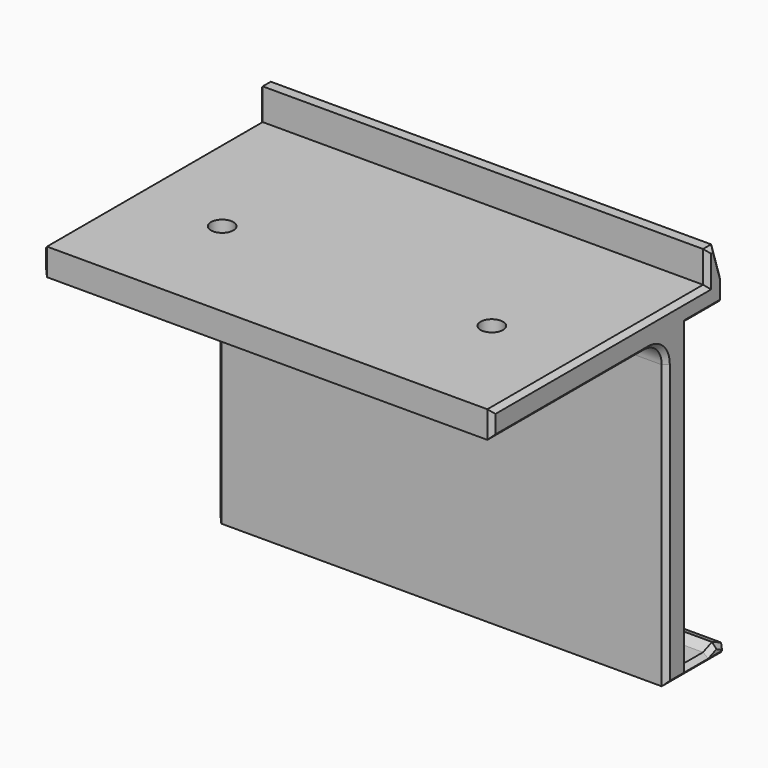
from build123d import *

# Parameters (mm, degrees)
F1_DEPTH = 50
F3_DEPTH = 100
F5_DEPTH = 100
F6_R     = 2.5
F7_DEPTH = 6
F8_R     = 5
F9_SIZE  = 0.99999


# Not quite as in the source:
# - a fillet or chamfer is up to 0.001 mm smaller than in the source, because OpenCascade refuses the exact size


with BuildPart() as f1:
    # F0 (on Right) → F1 (new body, symmetric)
    with BuildSketch(Plane.YZ):
        Polygon((0, 7), (0, 0), (-60, 0), (-60, -6), (-11.5, -6), (-11.5, -74), (5, -74), (5, -71), (0, -71), (0, -72), (-5.5, -72), (-5.5, -5), (4.5, -5), (4.5, 7), align=None)
    extrude(amount=F1_DEPTH, both=True)

    # F2 (on face) → F3 (cut, through all)
    with BuildSketch(Plane.YZ.offset(50)):
        Polygon((4.5, 7), (2.25, 7), (4.5, 0), align=None)
    extrude(amount=-F3_DEPTH, mode=Mode.SUBTRACT)

    # F4 (on face) → F5 (cut, through all)
    with BuildSketch(Plane.YZ.offset(50)):
        Polygon((0, -71), (0, -72), (2.5, -71), align=None)
        Polygon((5, -71), (2.5, -71), (5, -72.108708322), align=None)
    extrude(amount=-F5_DEPTH, mode=Mode.SUBTRACT)

    # F6 (on face) → F7 (cut, through all)
    with BuildSketch(Plane.XY):
        with Locations((-30, -35)):
            Circle(F6_R)
        with Locations((30, -35)):
            Circle(F6_R)
    extrude(amount=-F7_DEPTH, mode=Mode.SUBTRACT)

    # F8
    f8_edges = [f1.edges().sort_by_distance(p)[0] for p in [
        (0, -11.5, -6),
    ]]
    fillet(f8_edges, radius=F8_R)

    # F9 (size 1 in the source; OpenCascade refuses exactly that, so slightly less here)
    f9_edges = [f1.edges().sort_by_distance(p)[0] for p in [
        (50, -11.5, -42.5),
        (50, -12.964466, -7.464466),
        (50, -3.25, -74),
        (50, -38.25, -6),
        (50, 5, -73.054354),
        (50, -60, -3),
        (50, 3.75, -71.554354),
        (50, -30, 0),
        (50, 1.25, -71.5),
        (50, 0, 3.5),
        (50, -2.75, -72),
        (50, 1.125, 7),
        (50, -5.5, -38.5),
        (50, 3.375, 3.5),
        (50, -0.5, -5),
        (50, 4.5, -2.5),
        (-50, -11.5, -42.5),
        (-50, -12.964466, -7.464466),
        (-50, -3.25, -74),
        (-50, -38.25, -6),
        (-50, 5, -73.054354),
        (-50, -60, -3),
        (-50, 3.75, -71.554354),
        (-50, -30, 0),
        (-50, 1.25, -71.5),
        (-50, 0, 3.5),
        (-50, -2.75, -72),
        (-50, 1.125, 7),
        (-50, -5.5, -38.5),
        (-50, 3.375, 3.5),
        (-50, -0.5, -5),
        (-50, 4.5, -2.5),
    ]]
    chamfer(f9_edges, length=F9_SIZE)


solid = f1.part
